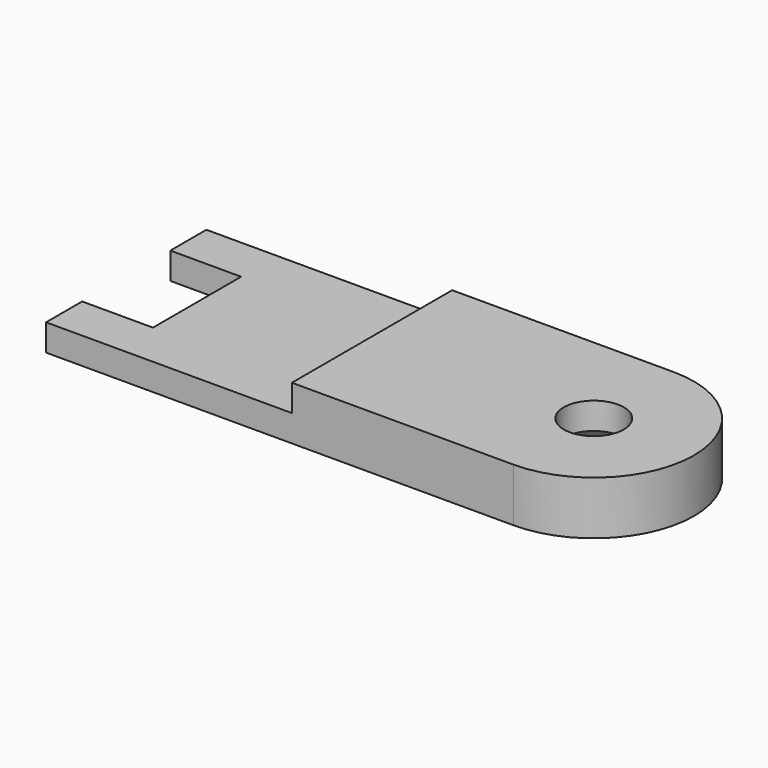
from build123d import *

# Parameters (mm, degrees)
F0_R     = 2.25
F1_DEPTH = 4
F2_DEPTH = 2
F3_SIZE  = 1.99999


# Not quite as in the source:
# - a fillet or chamfer is up to 0.001 mm smaller than in the source, because OpenCascade refuses the exact size


with BuildPart() as f1:
    # F0 (on Top) → F1 (new body)
    with BuildSketch(Plane.XY):
        with BuildLine():
            Line((14, 7.5), (-2.6, 7.5))
            Line((-2.6, 7.5), (-2.6, -7.5))
            Line((-2.6, -7.5), (14, -7.5))
            ThreePointArc((14, -7.5), (21.5, 0), (14, 7.5))
        make_face()
        with Locations((14, 0)):
            Circle(F0_R, mode=Mode.SUBTRACT)
    extrude(amount=F1_DEPTH)

    # F0 (on Top) → F2 (join)
    with BuildSketch(Plane.XY):
        Polygon((-2.6, 7.5), (-21, 7.5), (-21, 4.125), (-17.7, 4.125), (-17.7, -4.125), (-21, -4.125), (-21, -7.5), (-2.6, -7.5), align=None)
    extrude(amount=F2_DEPTH)

    # F3 (size 2 in the source; OpenCascade refuses exactly that, so slightly less here)
    f3_edges = [f1.edges().sort_by_distance(p)[0] for p in [
        (11.75, 0, 0),
        (-17.7, 0, 2),
    ]]
    chamfer(f3_edges, length=F3_SIZE)


solid = f1.part
